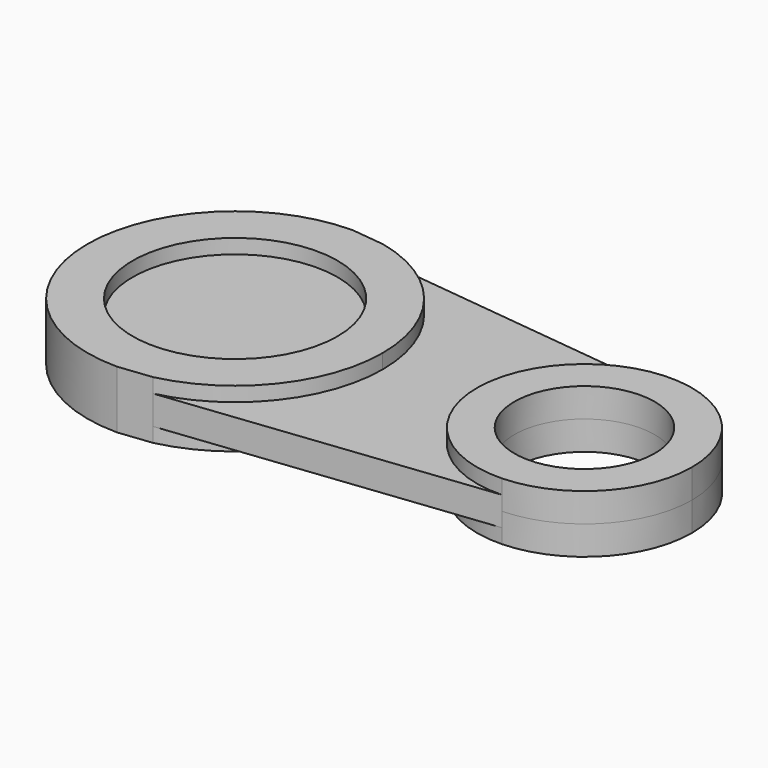
from build123d import *

# Parameters (mm, degrees)
F0_R     = 44.9480270959
F1_DEPTH = 12.7
F0_R_2   = 30.775716183
F2_DEPTH = 6.35


with BuildPart() as f1:
    # F0 (on Top) → F1 (new body, symmetric)
    with BuildSketch(Plane.XY):
        with BuildLine():
            Line((14.6048909022, 63.0824442065), (0, 64.751043276))
            ThreePointArc((0, 64.751043276), (-64.751043276, 0), (0, -64.751043276))
            Line((0, -64.751043276), (14.5651541935, -63.0916308923))
            ThreePointArc((14.5651541935, -63.0916308923), (50.6744833956, -40.3087377365), (64.751043276, 0))
            ThreePointArc((64.751043276, 0), (50.6871755387, 40.2927765392), (14.6048909022, 63.0824442065))
        make_face()
        Circle(F0_R, mode=Mode.SUBTRACT)
    extrude(amount=F1_DEPTH, both=True)


with BuildPart() as f1b:
    # F0 (on Top) → F1, piece 2 (new body, symmetric)
    with BuildSketch(Plane.XY):
        with BuildLine():
            ThreePointArc((200.4291468306, 0), (186.9360305833, 33.0180203257), (154.1803392628, 47.1360420854))
            ThreePointArc((154.1803392628, 47.1360420854), (106.1408512327, -0.2762262139), (154.7326209823, -47.1223093808))
            ThreePointArc((154.7326209823, -47.1223093808), (187.128909941, -32.8202853277), (200.4291468306, 0))
        make_face()
        with Locations((153.2845944166, 0)):
            Circle(F0_R_2, mode=Mode.SUBTRACT)
    extrude(amount=F1_DEPTH, both=True)


with BuildPart() as f2:
    # F0 (on Top) → F2 (new body, symmetric)
    with BuildSketch(Plane.XY):
        with BuildLine():
            Line((154.1803392628, 47.1360420854), (14.6048909022, 63.0824442065))
            ThreePointArc((14.6048909022, 63.0824442065), (50.6871755387, 40.2927765392), (64.751043276, 0))
            ThreePointArc((64.751043276, 0), (50.6744833956, -40.3087377365), (14.5651541935, -63.0916308923))
            Line((14.5651541935, -63.0916308923), (154.7326209823, -47.1223093808))
            ThreePointArc((154.7326209823, -47.1223093808), (106.1408512327, -0.2762262139), (154.1803392628, 47.1360420854))
        make_face()
    extrude(amount=F2_DEPTH, both=True)


with BuildPart() as f2b:
    # F0 (on Top) → F2, piece 2 (new body, symmetric)
    with BuildSketch(Plane.XY):
        Circle(F0_R)
    extrude(amount=F2_DEPTH, both=True)


solid = Compound([f1.part, f1b.part, f2.part, f2b.part])
